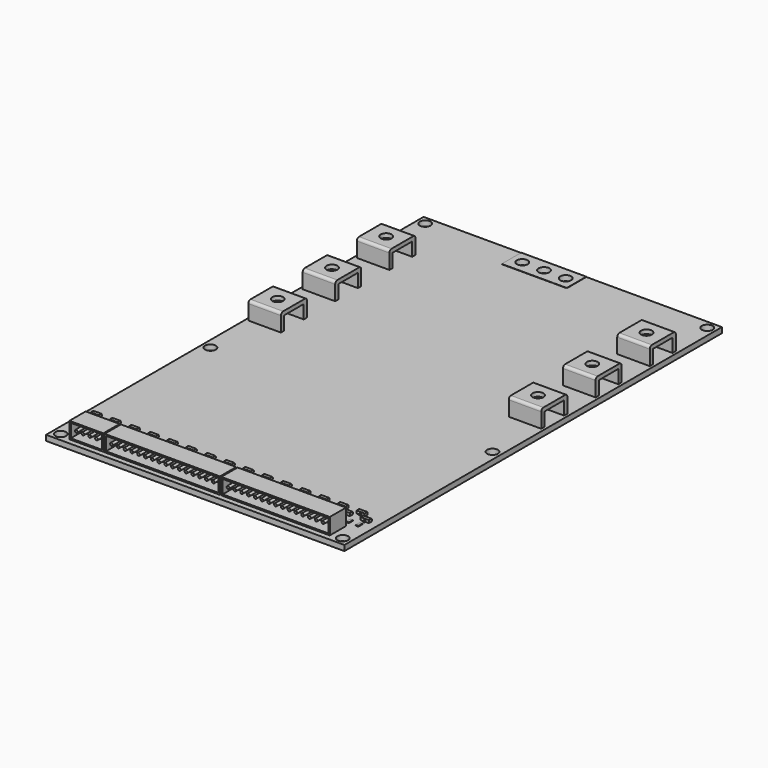
from build123d import *

# Parameters (mm, degrees)
F0_W      = 110
F0_H      = 174
F1_DEPTH  = 2
F3_D      = 4
F4_W      = 3
F4_H      = 1.2
F5_DEPTH  = 1
F6_W      = 0.45
F6_H      = 0.5
F7_DEPTH  = 0.5
F4_W_2    = 1
F8_DEPTH  = 0.25
F6_W_2    = 1
F6_H_2    = 1.2
F6_H_3    = 0.4
F9_DEPTH  = 0.25
F10_W     = 12.5
F10_H     = 7.5
F11_DEPTH = 6
F10_W_2   = 42.5
F10_W_3   = 40
F12_W     = 12
F12_H     = 12
F12_R     = 2
F13_DEPTH = 6.5
F14_W     = 9
F14_H     = 5
F15_DEPTH = 109.001
F16_R     = 1
F16_2_R   = 1
F16_3_R   = 1
F16_4_R   = 1
F16_5_R   = 1
F16_6_R   = 1
F17_W     = 24
F17_H     = 9
F17_R     = 2
F18_DEPTH = 0.1
F19_D     = 4.5
F19_DEPTH = 2.001
F20_W     = 39
F20_H     = 5
F20_R     = 0.5
F20_W_2   = 41.5
F20_W_3   = 11.5
F21_DEPTH = 5


with BuildPart() as f1:
    # F0 (on Top) → F1 (new body)
    with BuildSketch(Plane.XY):
        with Locations((25.1564069837, 32.1259858906)):
            Rectangle(F0_W, F0_H)
    extrude(amount=F1_DEPTH)

    # F3 (through all)
    with Locations(Plane.XY.offset(2)):
        with Locations((77.1564069837, 116.1259858906), (-26.8435930163, 116.1259858906), (-26.8435930163, 17.1259858906), (77.1564069837, 17.1259858906), (77.1564069837, -51.8740141094), (-26.8435930163, -51.8740141094)):
            Hole(F3_D / 2)

    # F19 (through all, one way)
    with BuildSketch(Plane.XY.offset(2)):
        with Locations((10.1564069837, 114.6259858906), (18.1564069837, 114.6259858906), (26.1564069837, 114.6259858906)):
            Circle(F19_D / 2)
    extrude(amount=-F19_DEPTH, mode=Mode.SUBTRACT)


with BuildPart() as f5:
    # F4 (on face) → F5 (new body)
    with BuildSketch(Plane.XY.offset(2)):
        with Locations((40.6564069837, -39.2740141094)):
            Rectangle(F4_W, F4_H)
    extrude(amount=F5_DEPTH)


with BuildPart() as f5b:
    # F4 (on face) → F5, piece 2 (new body)
    with BuildSketch(Plane.XY.offset(2)):
        with Locations((75.6564069837, -39.2740141094)):
            Rectangle(F4_W, F4_H)
    extrude(amount=F5_DEPTH)


with BuildPart() as f5c:
    # F4 (on face) → F5, piece 3 (new body)
    with BuildSketch(Plane.XY.offset(2)):
        with Locations((9.1564069837, -36.7740141094)):
            Rectangle(F4_W, F4_H)
    extrude(amount=F5_DEPTH)


with BuildPart() as f5d:
    # F4 (on face) → F5, piece 4 (new body)
    with BuildSketch(Plane.XY.offset(2)):
        with Locations((-11.8435930163, -36.7740141094)):
            Rectangle(F4_W, F4_H)
    extrude(amount=F5_DEPTH)


with BuildPart() as f5e:
    # F4 (on face) → F5, piece 5 (new body)
    with BuildSketch(Plane.XY.offset(2)):
        with Locations((23.1564069837, -36.7740141094)):
            Rectangle(F4_W, F4_H)
    extrude(amount=F5_DEPTH)


with BuildPart() as f5f:
    # F4 (on face) → F5, piece 6 (new body)
    with BuildSketch(Plane.XY.offset(2)):
        with Locations((-18.8435930163, -36.7740141094)):
            Rectangle(F4_W, F4_H)
    extrude(amount=F5_DEPTH)


with BuildPart() as f5g:
    # F4 (on face) → F5, piece 7 (new body)
    with BuildSketch(Plane.XY.offset(2)):
        with Locations((-1.3435930163, -39.2740141094)):
            Rectangle(F4_W, F4_H)
    extrude(amount=F5_DEPTH)


with BuildPart() as f5h:
    # F4 (on face) → F5, piece 8 (new body)
    with BuildSketch(Plane.XY.offset(2)):
        with Locations((12.6564069837, -39.2740141094)):
            Rectangle(F4_W, F4_H)
    extrude(amount=F5_DEPTH)


with BuildPart() as f5i:
    # F4 (on face) → F5, piece 9 (new body)
    with BuildSketch(Plane.XY.offset(2)):
        with Locations((51.1564069837, -36.7740141094)):
            Rectangle(F4_W, F4_H)
    extrude(amount=F5_DEPTH)


with BuildPart() as f5j:
    # F4 (on face) → F5, piece 10 (new body)
    with BuildSketch(Plane.XY.offset(2)):
        with Locations((72.1564069837, -36.7740141094)):
            Rectangle(F4_W, F4_H)
    extrude(amount=F5_DEPTH)


with BuildPart() as f5k:
    # F4 (on face) → F5, piece 11 (new body)
    with BuildSketch(Plane.XY.offset(2)):
        with Locations((-15.3435930163, -39.2740141094)):
            Rectangle(F4_W, F4_H)
    extrude(amount=F5_DEPTH)


with BuildPart() as f5l:
    # F4 (on face) → F5, piece 12 (new body)
    with BuildSketch(Plane.XY.offset(2)):
        with Locations((54.6564069837, -39.2740141094)):
            Rectangle(F4_W, F4_H)
    extrude(amount=F5_DEPTH)


with BuildPart() as f5m:
    # F4 (on face) → F5, piece 13 (new body)
    with BuildSketch(Plane.XY.offset(2)):
        with Locations((68.6564069837, -39.2740141094)):
            Rectangle(F4_W, F4_H)
    extrude(amount=F5_DEPTH)


with BuildPart() as f5n:
    # F4 (on face) → F5, piece 14 (new body)
    with BuildSketch(Plane.XY.offset(2)):
        with Locations((26.6564069837, -39.2740141094)):
            Rectangle(F4_W, F4_H)
    extrude(amount=F5_DEPTH)


with BuildPart() as f5o:
    # F4 (on face) → F5, piece 15 (new body)
    with BuildSketch(Plane.XY.offset(2)):
        with Locations((44.1564069837, -36.7740141094)):
            Rectangle(F4_W, F4_H)
    extrude(amount=F5_DEPTH)


with BuildPart() as f5p:
    # F4 (on face) → F5, piece 16 (new body)
    with BuildSketch(Plane.XY.offset(2)):
        with Locations((37.1564069837, -36.7740141094)):
            Rectangle(F4_W, F4_H)
    extrude(amount=F5_DEPTH)


with BuildPart() as f5q:
    # F4 (on face) → F5, piece 17 (new body)
    with BuildSketch(Plane.XY.offset(2)):
        with Locations((-22.3435930163, -39.2740141094)):
            Rectangle(F4_W, F4_H)
    extrude(amount=F5_DEPTH)


with BuildPart() as f5r:
    # F4 (on face) → F5, piece 18 (new body)
    with BuildSketch(Plane.XY.offset(2)):
        with Locations((5.6564069837, -39.2740141094)):
            Rectangle(F4_W, F4_H)
    extrude(amount=F5_DEPTH)


with BuildPart() as f5s:
    # F4 (on face) → F5, piece 19 (new body)
    with BuildSketch(Plane.XY.offset(2)):
        with Locations((16.1564069837, -36.7740141094)):
            Rectangle(F4_W, F4_H)
    extrude(amount=F5_DEPTH)


with BuildPart() as f5t:
    # F4 (on face) → F5, piece 20 (new body)
    with BuildSketch(Plane.XY.offset(2)):
        with Locations((-4.8435930163, -36.7740141094)):
            Rectangle(F4_W, F4_H)
    extrude(amount=F5_DEPTH)


with BuildPart() as f5u:
    # F4 (on face) → F5, piece 21 (new body)
    with BuildSketch(Plane.XY.offset(2)):
        with Locations((33.6564069837, -39.2740141094)):
            Rectangle(F4_W, F4_H)
    extrude(amount=F5_DEPTH)


with BuildPart() as f5v:
    # F4 (on face) → F5, piece 22 (new body)
    with BuildSketch(Plane.XY.offset(2)):
        with Locations((47.6564069837, -39.2740141094)):
            Rectangle(F4_W, F4_H)
    extrude(amount=F5_DEPTH)


with BuildPart() as f5w:
    # F4 (on face) → F5, piece 23 (new body)
    with BuildSketch(Plane.XY.offset(2)):
        with Locations((61.6564069837, -39.2740141094)):
            Rectangle(F4_W, F4_H)
    extrude(amount=F5_DEPTH)


with BuildPart() as f5x:
    # F4 (on face) → F5, piece 24 (new body)
    with BuildSketch(Plane.XY.offset(2)):
        with Locations((19.6564069837, -39.2740141094)):
            Rectangle(F4_W, F4_H)
    extrude(amount=F5_DEPTH)


with BuildPart() as f5y:
    # F4 (on face) → F5, piece 25 (new body)
    with BuildSketch(Plane.XY.offset(2)):
        with Locations((58.1564069837, -36.7740141094)):
            Rectangle(F4_W, F4_H)
    extrude(amount=F5_DEPTH)


with BuildPart() as f5z:
    # F4 (on face) → F5, piece 26 (new body)
    with BuildSketch(Plane.XY.offset(2)):
        with Locations((65.1564069837, -36.7740141094)):
            Rectangle(F4_W, F4_H)
    extrude(amount=F5_DEPTH)


with BuildPart() as f5ba:
    # F4 (on face) → F5, piece 27 (new body)
    with BuildSketch(Plane.XY.offset(2)):
        with Locations((-8.3435930163, -39.2740141094)):
            Rectangle(F4_W, F4_H)
    extrude(amount=F5_DEPTH)


with BuildPart() as f5bb:
    # F4 (on face) → F5, piece 28 (new body)
    with BuildSketch(Plane.XY.offset(2)):
        with Locations((-25.8435930163, -36.7740141094)):
            Rectangle(F4_W, F4_H)
    extrude(amount=F5_DEPTH)


with BuildPart() as f5bc:
    # F4 (on face) → F5, piece 29 (new body)
    with BuildSketch(Plane.XY.offset(2)):
        with Locations((30.1564069837, -36.7740141094)):
            Rectangle(F4_W, F4_H)
    extrude(amount=F5_DEPTH)


with BuildPart() as f5bd:
    # F4 (on face) → F5, piece 30 (new body)
    with BuildSketch(Plane.XY.offset(2)):
        with Locations((2.1564069837, -36.7740141094)):
            Rectangle(F4_W, F4_H)
    extrude(amount=F5_DEPTH)


with BuildPart() as f7:
    # F6 (on face) → F7 (new body)
    with BuildSketch(Plane.XY.offset(2)):
        with Locations((12.6564069837, -40.1240141094)):
            Rectangle(F6_W, F6_H)
        with Locations((-0.3435930163, -38.4240141094)):
            Rectangle(F6_W, F6_H)
        with Locations((52.1564069837, -35.9240141094)):
            Rectangle(F6_W, F6_H)
        with Locations((74.6564069837, -38.4240141094)):
            Rectangle(F6_W, F6_H)
        with Locations((67.6564069837, -38.4240141094)):
            Rectangle(F6_W, F6_H)
        with Locations((25.6564069837, -38.4240141094)):
            Rectangle(F6_W, F6_H)
        with Locations((71.1564069837, -35.9240141094)):
            Rectangle(F6_W, F6_H)
        with Locations((-15.3435930163, -40.1240141094)):
            Rectangle(F6_W, F6_H)
        with Locations((15.1564069837, -35.9240141094)):
            Rectangle(F6_W, F6_H)
        with Locations((-23.3435930163, -38.4240141094)):
            Rectangle(F6_W, F6_H)
        with Locations((13.6564069837, -38.4240141094)):
            Rectangle(F6_W, F6_H)
        with Locations((-5.8435930163, -35.9240141094)):
            Rectangle(F6_W, F6_H)
        with Locations((27.6564069837, -38.4240141094)):
            Rectangle(F6_W, F6_H)
        with Locations((43.1564069837, -35.9240141094)):
            Rectangle(F6_W, F6_H)
        with Locations((41.6564069837, -38.4240141094)):
            Rectangle(F6_W, F6_H)
        with Locations((-10.8435930163, -35.9240141094)):
            Rectangle(F6_W, F6_H)
        with Locations((-19.8435930163, -35.9240141094)):
            Rectangle(F6_W, F6_H)
        with Locations((44.1564069837, -37.6240141094)):
            Rectangle(F6_W, F6_H)
        with Locations((20.6564069837, -38.4240141094)):
            Rectangle(F6_W, F6_H)
        with Locations((46.6564069837, -38.4240141094)):
            Rectangle(F6_W, F6_H)
        with Locations((-2.3435930163, -38.4240141094)):
            Rectangle(F6_W, F6_H)
        with Locations((-8.3435930163, -40.1240141094)):
            Rectangle(F6_W, F6_H)
        with Locations((-18.8435930163, -37.6240141094)):
            Rectangle(F6_W, F6_H)
        with Locations((-1.3435930163, -40.1240141094)):
            Rectangle(F6_W, F6_H)
        with Locations((32.6564069837, -38.4240141094)):
            Rectangle(F6_W, F6_H)
        with Locations((66.1564069837, -35.9240141094)):
            Rectangle(F6_W, F6_H)
        with Locations((16.1564069837, -37.6240141094)):
            Rectangle(F6_W, F6_H)
        with Locations((26.6564069837, -40.1240141094)):
            Rectangle(F6_W, F6_H)
        with Locations((50.1564069837, -35.9240141094)):
            Rectangle(F6_W, F6_H)
        with Locations((24.1564069837, -35.9240141094)):
            Rectangle(F6_W, F6_H)
        with Locations((36.1564069837, -35.9240141094)):
            Rectangle(F6_W, F6_H)
        with Locations((37.1564069837, -37.6240141094)):
            Rectangle(F6_W, F6_H)
        with Locations((34.6564069837, -38.4240141094)):
            Rectangle(F6_W, F6_H)
        with Locations((53.6564069837, -38.4240141094)):
            Rectangle(F6_W, F6_H)
        with Locations((55.6564069837, -38.4240141094)):
            Rectangle(F6_W, F6_H)
        with Locations((-3.8435930163, -35.9240141094)):
            Rectangle(F6_W, F6_H)
        with Locations((17.1564069837, -35.9240141094)):
            Rectangle(F6_W, F6_H)
        with Locations((-21.3435930163, -38.4240141094)):
            Rectangle(F6_W, F6_H)
        with Locations((54.6564069837, -40.1240141094)):
            Rectangle(F6_W, F6_H)
        with Locations((68.6564069837, -40.1240141094)):
            Rectangle(F6_W, F6_H)
        with Locations((-7.3435930163, -38.4240141094)):
            Rectangle(F6_W, F6_H)
        with Locations((40.6564069837, -40.1240141094)):
            Rectangle(F6_W, F6_H)
        with Locations((62.6564069837, -38.4240141094)):
            Rectangle(F6_W, F6_H)
        with Locations((29.1564069837, -35.9240141094)):
            Rectangle(F6_W, F6_H)
        with Locations((-4.8435930163, -37.6240141094)):
            Rectangle(F6_W, F6_H)
        with Locations((64.1564069837, -35.9240141094)):
            Rectangle(F6_W, F6_H)
        with Locations((8.1564069837, -35.9240141094)):
            Rectangle(F6_W, F6_H)
        with Locations((48.6564069837, -38.4240141094)):
            Rectangle(F6_W, F6_H)
        with Locations((-17.8435930163, -35.9240141094)):
            Rectangle(F6_W, F6_H)
        with Locations((38.1564069837, -35.9240141094)):
            Rectangle(F6_W, F6_H)
        with Locations((69.6564069837, -38.4240141094)):
            Rectangle(F6_W, F6_H)
        with Locations((10.1564069837, -35.9240141094)):
            Rectangle(F6_W, F6_H)
        with Locations((-26.8435930163, -35.9240141094)):
            Rectangle(F6_W, F6_H)
        with Locations((57.1564069837, -35.9240141094)):
            Rectangle(F6_W, F6_H)
        with Locations((76.6564069837, -38.4240141094)):
            Rectangle(F6_W, F6_H)
        with Locations((39.6564069837, -38.4240141094)):
            Rectangle(F6_W, F6_H)
        with Locations((65.1564069837, -37.6240141094)):
            Rectangle(F6_W, F6_H)
        with Locations((11.6564069837, -38.4240141094)):
            Rectangle(F6_W, F6_H)
        with Locations((23.1564069837, -37.6240141094)):
            Rectangle(F6_W, F6_H)
        with Locations((1.1564069837, -35.9240141094)):
            Rectangle(F6_W, F6_H)
        with Locations((51.1564069837, -37.6240141094)):
            Rectangle(F6_W, F6_H)
        with Locations((22.1564069837, -35.9240141094)):
            Rectangle(F6_W, F6_H)
        with Locations((-12.8435930163, -35.9240141094)):
            Rectangle(F6_W, F6_H)
        with Locations((9.1564069837, -37.6240141094)):
            Rectangle(F6_W, F6_H)
        with Locations((19.6564069837, -40.1240141094)):
            Rectangle(F6_W, F6_H)
        with Locations((6.6564069837, -38.4240141094)):
            Rectangle(F6_W, F6_H)
        with Locations((-16.3435930163, -38.4240141094)):
            Rectangle(F6_W, F6_H)
        with Locations((-22.3435930163, -40.1240141094)):
            Rectangle(F6_W, F6_H)
        with Locations((-14.3435930163, -38.4240141094)):
            Rectangle(F6_W, F6_H)
        with Locations((75.6564069837, -40.1240141094)):
            Rectangle(F6_W, F6_H)
        with Locations((73.1564069837, -35.9240141094)):
            Rectangle(F6_W, F6_H)
        with Locations((2.1564069837, -37.6240141094)):
            Rectangle(F6_W, F6_H)
        with Locations((45.1564069837, -35.9240141094)):
            Rectangle(F6_W, F6_H)
        with Locations((-24.8435930163, -35.9240141094)):
            Rectangle(F6_W, F6_H)
        with Locations((58.1564069837, -37.6240141094)):
            Rectangle(F6_W, F6_H)
        with Locations((18.6564069837, -38.4240141094)):
            Rectangle(F6_W, F6_H)
        with Locations((47.6564069837, -40.1240141094)):
            Rectangle(F6_W, F6_H)
        with Locations((33.6564069837, -40.1240141094)):
            Rectangle(F6_W, F6_H)
        with Locations((31.1564069837, -35.9240141094)):
            Rectangle(F6_W, F6_H)
        with Locations((30.1564069837, -37.6240141094)):
            Rectangle(F6_W, F6_H)
        with Locations((-25.8435930163, -37.6240141094)):
            Rectangle(F6_W, F6_H)
        with Locations((60.6564069837, -38.4240141094)):
            Rectangle(F6_W, F6_H)
        with Locations((-9.3435930163, -38.4240141094)):
            Rectangle(F6_W, F6_H)
        with Locations((61.6564069837, -40.1240141094)):
            Rectangle(F6_W, F6_H)
        with Locations((-11.8435930163, -37.6240141094)):
            Rectangle(F6_W, F6_H)
        with Locations((3.1564069837, -35.9240141094)):
            Rectangle(F6_W, F6_H)
        with Locations((5.6564069837, -40.1240141094)):
            Rectangle(F6_W, F6_H)
        with Locations((59.1564069837, -35.9240141094)):
            Rectangle(F6_W, F6_H)
        with Locations((4.6564069837, -38.4240141094)):
            Rectangle(F6_W, F6_H)
        with Locations((72.1564069837, -37.6240141094)):
            Rectangle(F6_W, F6_H)
    extrude(amount=F7_DEPTH)


with BuildPart() as f8:
    # F4 (on face) → F8 (new body)
    with BuildSketch(Plane.XY.offset(2)):
        with Locations((-18.8435930163, -42.4740141094)):
            Rectangle(F4_W_2, F4_H)
    extrude(amount=F8_DEPTH)


with BuildPart() as f8b:
    # F4 (on face) → F8, piece 2 (new body)
    with BuildSketch(Plane.XY.offset(2)):
        with Locations((-22.3435930163, -42.4740141094)):
            Rectangle(F4_W_2, F4_H)
    extrude(amount=F8_DEPTH)


with BuildPart() as f8c:
    # F4 (on face) → F8, piece 3 (new body)
    with BuildSketch(Plane.XY.offset(2)):
        with Locations((26.6564069837, -42.4740141094)):
            Rectangle(F4_W_2, F4_H)
    extrude(amount=F8_DEPTH)


with BuildPart() as f8d:
    # F4 (on face) → F8, piece 4 (new body)
    with BuildSketch(Plane.XY.offset(2)):
        with Locations((-25.8435930163, -42.4740141094)):
            Rectangle(F4_W_2, F4_H)
    extrude(amount=F8_DEPTH)


with BuildPart() as f8e:
    # F4 (on face) → F8, piece 5 (new body)
    with BuildSketch(Plane.XY.offset(2)):
        with Locations((51.1564069837, -42.4740141094)):
            Rectangle(F4_W_2, F4_H)
    extrude(amount=F8_DEPTH)


with BuildPart() as f8f:
    # F4 (on face) → F8, piece 6 (new body)
    with BuildSketch(Plane.XY.offset(2)):
        with Locations((44.1564069837, -42.4740141094)):
            Rectangle(F4_W_2, F4_H)
    extrude(amount=F8_DEPTH)


with BuildPart() as f8g:
    # F4 (on face) → F8, piece 7 (new body)
    with BuildSketch(Plane.XY.offset(2)):
        with Locations((65.1564069837, -42.4740141094)):
            Rectangle(F4_W_2, F4_H)
    extrude(amount=F8_DEPTH)


with BuildPart() as f8h:
    # F4 (on face) → F8, piece 8 (new body)
    with BuildSketch(Plane.XY.offset(2)):
        with Locations((61.6564069837, -42.4740141094)):
            Rectangle(F4_W_2, F4_H)
    extrude(amount=F8_DEPTH)


with BuildPart() as f8i:
    # F4 (on face) → F8, piece 9 (new body)
    with BuildSketch(Plane.XY.offset(2)):
        with Locations((40.6564069837, -42.4740141094)):
            Rectangle(F4_W_2, F4_H)
    extrude(amount=F8_DEPTH)


with BuildPart() as f8j:
    # F4 (on face) → F8, piece 10 (new body)
    with BuildSketch(Plane.XY.offset(2)):
        with Locations((33.6564069837, -42.4740141094)):
            Rectangle(F4_W_2, F4_H)
    extrude(amount=F8_DEPTH)


with BuildPart() as f8k:
    # F4 (on face) → F8, piece 11 (new body)
    with BuildSketch(Plane.XY.offset(2)):
        with Locations((75.6564069837, -42.4740141094)):
            Rectangle(F4_W_2, F4_H)
    extrude(amount=F8_DEPTH)


with BuildPart() as f8l:
    # F4 (on face) → F8, piece 12 (new body)
    with BuildSketch(Plane.XY.offset(2)):
        with Locations((54.6564069837, -42.4740141094)):
            Rectangle(F4_W_2, F4_H)
    extrude(amount=F8_DEPTH)


with BuildPart() as f8m:
    # F4 (on face) → F8, piece 13 (new body)
    with BuildSketch(Plane.XY.offset(2)):
        with Locations((47.6564069837, -42.4740141094)):
            Rectangle(F4_W_2, F4_H)
    extrude(amount=F8_DEPTH)


with BuildPart() as f8n:
    # F4 (on face) → F8, piece 14 (new body)
    with BuildSketch(Plane.XY.offset(2)):
        with Locations((-15.3435930163, -42.4740141094)):
            Rectangle(F4_W_2, F4_H)
    extrude(amount=F8_DEPTH)


with BuildPart() as f8o:
    # F4 (on face) → F8, piece 15 (new body)
    with BuildSketch(Plane.XY.offset(2)):
        with Locations((12.6564069837, -42.4740141094)):
            Rectangle(F4_W_2, F4_H)
    extrude(amount=F8_DEPTH)


with BuildPart() as f8p:
    # F4 (on face) → F8, piece 16 (new body)
    with BuildSketch(Plane.XY.offset(2)):
        with Locations((-8.3435930163, -42.4740141094)):
            Rectangle(F4_W_2, F4_H)
    extrude(amount=F8_DEPTH)


with BuildPart() as f8q:
    # F4 (on face) → F8, piece 17 (new body)
    with BuildSketch(Plane.XY.offset(2)):
        with Locations((-1.3435930163, -42.4740141094)):
            Rectangle(F4_W_2, F4_H)
    extrude(amount=F8_DEPTH)


with BuildPart() as f8r:
    # F4 (on face) → F8, piece 18 (new body)
    with BuildSketch(Plane.XY.offset(2)):
        with Locations((19.6564069837, -42.4740141094)):
            Rectangle(F4_W_2, F4_H)
    extrude(amount=F8_DEPTH)


with BuildPart() as f8s:
    # F4 (on face) → F8, piece 19 (new body)
    with BuildSketch(Plane.XY.offset(2)):
        with Locations((5.6564069837, -42.4740141094)):
            Rectangle(F4_W_2, F4_H)
    extrude(amount=F8_DEPTH)


with BuildPart() as f8t:
    # F4 (on face) → F8, piece 20 (new body)
    with BuildSketch(Plane.XY.offset(2)):
        with Locations((72.1564069837, -42.4740141094)):
            Rectangle(F4_W_2, F4_H)
    extrude(amount=F8_DEPTH)


with BuildPart() as f8u:
    # F4 (on face) → F8, piece 21 (new body)
    with BuildSketch(Plane.XY.offset(2)):
        with Locations((58.1564069837, -42.4740141094)):
            Rectangle(F4_W_2, F4_H)
    extrude(amount=F8_DEPTH)


with BuildPart() as f8v:
    # F4 (on face) → F8, piece 22 (new body)
    with BuildSketch(Plane.XY.offset(2)):
        with Locations((30.1564069837, -42.4740141094)):
            Rectangle(F4_W_2, F4_H)
    extrude(amount=F8_DEPTH)


with BuildPart() as f8w:
    # F4 (on face) → F8, piece 23 (new body)
    with BuildSketch(Plane.XY.offset(2)):
        with Locations((9.1564069837, -42.4740141094)):
            Rectangle(F4_W_2, F4_H)
    extrude(amount=F8_DEPTH)


with BuildPart() as f8x:
    # F4 (on face) → F8, piece 24 (new body)
    with BuildSketch(Plane.XY.offset(2)):
        with Locations((-11.8435930163, -42.4740141094)):
            Rectangle(F4_W_2, F4_H)
    extrude(amount=F8_DEPTH)


with BuildPart() as f8y:
    # F4 (on face) → F8, piece 25 (new body)
    with BuildSketch(Plane.XY.offset(2)):
        with Locations((-4.8435930163, -42.4740141094)):
            Rectangle(F4_W_2, F4_H)
    extrude(amount=F8_DEPTH)


with BuildPart() as f8z:
    # F4 (on face) → F8, piece 26 (new body)
    with BuildSketch(Plane.XY.offset(2)):
        with Locations((16.1564069837, -42.4740141094)):
            Rectangle(F4_W_2, F4_H)
    extrude(amount=F8_DEPTH)


with BuildPart() as f8ba:
    # F4 (on face) → F8, piece 27 (new body)
    with BuildSketch(Plane.XY.offset(2)):
        with Locations((23.1564069837, -42.4740141094)):
            Rectangle(F4_W_2, F4_H)
    extrude(amount=F8_DEPTH)


with BuildPart() as f8bb:
    # F4 (on face) → F8, piece 28 (new body)
    with BuildSketch(Plane.XY.offset(2)):
        with Locations((2.1564069837, -42.4740141094)):
            Rectangle(F4_W_2, F4_H)
    extrude(amount=F8_DEPTH)


with BuildPart() as f8bc:
    # F4 (on face) → F8, piece 29 (new body)
    with BuildSketch(Plane.XY.offset(2)):
        with Locations((68.6564069837, -42.4740141094)):
            Rectangle(F4_W_2, F4_H)
    extrude(amount=F8_DEPTH)


with BuildPart() as f8bd:
    # F4 (on face) → F8, piece 30 (new body)
    with BuildSketch(Plane.XY.offset(2)):
        with Locations((37.1564069837, -42.4740141094)):
            Rectangle(F4_W_2, F4_H)
    extrude(amount=F8_DEPTH)


with BuildPart() as f8be:
    # F6 (on face) → F8, piece 31 (new body)
    with BuildSketch(Plane.XY.offset(2)):
        with Locations((2.1564069837, -42.4740141094)):
            Rectangle(F6_W_2, F6_H_2)
    extrude(amount=F8_DEPTH)


with BuildPart() as f8bf:
    # F6 (on face) → F8, piece 32 (new body)
    with BuildSketch(Plane.XY.offset(2)):
        with Locations((33.6564069837, -42.4740141094)):
            Rectangle(F6_W_2, F6_H_2)
    extrude(amount=F8_DEPTH)


with BuildPart() as f8bg:
    # F6 (on face) → F8, piece 33 (new body)
    with BuildSketch(Plane.XY.offset(2)):
        with Locations((-1.3435930163, -42.4740141094)):
            Rectangle(F6_W_2, F6_H_2)
    extrude(amount=F8_DEPTH)


with BuildPart() as f8bh:
    # F6 (on face) → F8, piece 34 (new body)
    with BuildSketch(Plane.XY.offset(2)):
        with Locations((23.1564069837, -42.4740141094)):
            Rectangle(F6_W_2, F6_H_2)
    extrude(amount=F8_DEPTH)


with BuildPart() as f8bi:
    # F6 (on face) → F8, piece 35 (new body)
    with BuildSketch(Plane.XY.offset(2)):
        with Locations((16.1564069837, -42.4740141094)):
            Rectangle(F6_W_2, F6_H_2)
    extrude(amount=F8_DEPTH)


with BuildPart() as f8bj:
    # F6 (on face) → F8, piece 36 (new body)
    with BuildSketch(Plane.XY.offset(2)):
        with Locations((5.6564069837, -42.4740141094)):
            Rectangle(F6_W_2, F6_H_2)
    extrude(amount=F8_DEPTH)


with BuildPart() as f8bk:
    # F6 (on face) → F8, piece 37 (new body)
    with BuildSketch(Plane.XY.offset(2)):
        with Locations((54.6564069837, -42.4740141094)):
            Rectangle(F6_W_2, F6_H_2)
    extrude(amount=F8_DEPTH)


with BuildPart() as f8bl:
    # F6 (on face) → F8, piece 38 (new body)
    with BuildSketch(Plane.XY.offset(2)):
        with Locations((30.1564069837, -42.4740141094)):
            Rectangle(F6_W_2, F6_H_2)
    extrude(amount=F8_DEPTH)


with BuildPart() as f8bm:
    # F6 (on face) → F8, piece 39 (new body)
    with BuildSketch(Plane.XY.offset(2)):
        with Locations((-22.3435930163, -42.4740141094)):
            Rectangle(F6_W_2, F6_H_2)
    extrude(amount=F8_DEPTH)


with BuildPart() as f8bn:
    # F6 (on face) → F8, piece 40 (new body)
    with BuildSketch(Plane.XY.offset(2)):
        with Locations((68.6564069837, -42.4740141094)):
            Rectangle(F6_W_2, F6_H_2)
    extrude(amount=F8_DEPTH)


with BuildPart() as f8bo:
    # F6 (on face) → F8, piece 41 (new body)
    with BuildSketch(Plane.XY.offset(2)):
        with Locations((-18.8435930163, -42.4740141094)):
            Rectangle(F6_W_2, F6_H_2)
    extrude(amount=F8_DEPTH)


with BuildPart() as f8bp:
    # F6 (on face) → F8, piece 42 (new body)
    with BuildSketch(Plane.XY.offset(2)):
        with Locations((-15.3435930163, -42.4740141094)):
            Rectangle(F6_W_2, F6_H_2)
    extrude(amount=F8_DEPTH)


with BuildPart() as f8bq:
    # F6 (on face) → F8, piece 43 (new body)
    with BuildSketch(Plane.XY.offset(2)):
        with Locations((37.1564069837, -42.4740141094)):
            Rectangle(F6_W_2, F6_H_2)
    extrude(amount=F8_DEPTH)


with BuildPart() as f8br:
    # F6 (on face) → F8, piece 44 (new body)
    with BuildSketch(Plane.XY.offset(2)):
        with Locations((-25.8435930163, -42.4740141094)):
            Rectangle(F6_W_2, F6_H_2)
    extrude(amount=F8_DEPTH)


with BuildPart() as f8bs:
    # F6 (on face) → F8, piece 45 (new body)
    with BuildSketch(Plane.XY.offset(2)):
        with Locations((19.6564069837, -42.4740141094)):
            Rectangle(F6_W_2, F6_H_2)
    extrude(amount=F8_DEPTH)


with BuildPart() as f8bt:
    # F6 (on face) → F8, piece 46 (new body)
    with BuildSketch(Plane.XY.offset(2)):
        with Locations((26.6564069837, -42.4740141094)):
            Rectangle(F6_W_2, F6_H_2)
    extrude(amount=F8_DEPTH)


with BuildPart() as f8bu:
    # F6 (on face) → F8, piece 47 (new body)
    with BuildSketch(Plane.XY.offset(2)):
        with Locations((75.6564069837, -42.4740141094)):
            Rectangle(F6_W_2, F6_H_2)
    extrude(amount=F8_DEPTH)


with BuildPart() as f8bv:
    # F6 (on face) → F8, piece 48 (new body)
    with BuildSketch(Plane.XY.offset(2)):
        with Locations((-4.8435930163, -42.4740141094)):
            Rectangle(F6_W_2, F6_H_2)
    extrude(amount=F8_DEPTH)


with BuildPart() as f8bw:
    # F6 (on face) → F8, piece 49 (new body)
    with BuildSketch(Plane.XY.offset(2)):
        with Locations((58.1564069837, -42.4740141094)):
            Rectangle(F6_W_2, F6_H_2)
    extrude(amount=F8_DEPTH)


with BuildPart() as f8bx:
    # F6 (on face) → F8, piece 50 (new body)
    with BuildSketch(Plane.XY.offset(2)):
        with Locations((40.6564069837, -42.4740141094)):
            Rectangle(F6_W_2, F6_H_2)
    extrude(amount=F8_DEPTH)


with BuildPart() as f8by:
    # F6 (on face) → F8, piece 51 (new body)
    with BuildSketch(Plane.XY.offset(2)):
        with Locations((72.1564069837, -42.4740141094)):
            Rectangle(F6_W_2, F6_H_2)
    extrude(amount=F8_DEPTH)


with BuildPart() as f8bz:
    # F6 (on face) → F8, piece 52 (new body)
    with BuildSketch(Plane.XY.offset(2)):
        with Locations((9.1564069837, -42.4740141094)):
            Rectangle(F6_W_2, F6_H_2)
    extrude(amount=F8_DEPTH)


with BuildPart() as f8ca:
    # F6 (on face) → F8, piece 53 (new body)
    with BuildSketch(Plane.XY.offset(2)):
        with Locations((65.1564069837, -42.4740141094)):
            Rectangle(F6_W_2, F6_H_2)
    extrude(amount=F8_DEPTH)


with BuildPart() as f8cb:
    # F6 (on face) → F8, piece 54 (new body)
    with BuildSketch(Plane.XY.offset(2)):
        with Locations((44.1564069837, -42.4740141094)):
            Rectangle(F6_W_2, F6_H_2)
    extrude(amount=F8_DEPTH)


with BuildPart() as f8cc:
    # F6 (on face) → F8, piece 55 (new body)
    with BuildSketch(Plane.XY.offset(2)):
        with Locations((12.6564069837, -42.4740141094)):
            Rectangle(F6_W_2, F6_H_2)
    extrude(amount=F8_DEPTH)


with BuildPart() as f8cd:
    # F6 (on face) → F8, piece 56 (new body)
    with BuildSketch(Plane.XY.offset(2)):
        with Locations((61.6564069837, -42.4740141094)):
            Rectangle(F6_W_2, F6_H_2)
    extrude(amount=F8_DEPTH)


with BuildPart() as f8ce:
    # F6 (on face) → F8, piece 57 (new body)
    with BuildSketch(Plane.XY.offset(2)):
        with Locations((-11.8435930163, -42.4740141094)):
            Rectangle(F6_W_2, F6_H_2)
    extrude(amount=F8_DEPTH)


with BuildPart() as f8cf:
    # F6 (on face) → F8, piece 58 (new body)
    with BuildSketch(Plane.XY.offset(2)):
        with Locations((47.6564069837, -42.4740141094)):
            Rectangle(F6_W_2, F6_H_2)
    extrude(amount=F8_DEPTH)


with BuildPart() as f8cg:
    # F6 (on face) → F8, piece 59 (new body)
    with BuildSketch(Plane.XY.offset(2)):
        with Locations((51.1564069837, -42.4740141094)):
            Rectangle(F6_W_2, F6_H_2)
    extrude(amount=F8_DEPTH)


with BuildPart() as f8ch:
    # F6 (on face) → F8, piece 60 (new body)
    with BuildSketch(Plane.XY.offset(2)):
        with Locations((-8.3435930163, -42.4740141094)):
            Rectangle(F6_W_2, F6_H_2)
    extrude(amount=F8_DEPTH)


with BuildPart() as f9:
    # F6 (on face) → F9 (new body)
    with BuildSketch(Plane.XY.offset(2)):
        with Locations((54.6564069837, -41.6740141094)):
            Rectangle(F6_W_2, F6_H_3)
    extrude(amount=F9_DEPTH)


with BuildPart() as f9b:
    # F6 (on face) → F9, piece 2 (new body)
    with BuildSketch(Plane.XY.offset(2)):
        with Locations((26.6564069837, -41.6740141094)):
            Rectangle(F6_W_2, F6_H_3)
    extrude(amount=F9_DEPTH)


with BuildPart() as f9c:
    # F6 (on face) → F9, piece 3 (new body)
    with BuildSketch(Plane.XY.offset(2)):
        with Locations((-1.3435930163, -41.6740141094)):
            Rectangle(F6_W_2, F6_H_3)
    extrude(amount=F9_DEPTH)


with BuildPart() as f9d:
    # F6 (on face) → F9, piece 4 (new body)
    with BuildSketch(Plane.XY.offset(2)):
        with Locations((33.6564069837, -41.6740141094)):
            Rectangle(F6_W_2, F6_H_3)
    extrude(amount=F9_DEPTH)


with BuildPart() as f9e:
    # F6 (on face) → F9, piece 5 (new body)
    with BuildSketch(Plane.XY.offset(2)):
        with Locations((37.1564069837, -41.6740141094)):
            Rectangle(F6_W_2, F6_H_3)
    extrude(amount=F9_DEPTH)


with BuildPart() as f9f:
    # F6 (on face) → F9, piece 6 (new body)
    with BuildSketch(Plane.XY.offset(2)):
        with Locations((23.1564069837, -41.6740141094)):
            Rectangle(F6_W_2, F6_H_3)
    extrude(amount=F9_DEPTH)


with BuildPart() as f9g:
    # F6 (on face) → F9, piece 7 (new body)
    with BuildSketch(Plane.XY.offset(2)):
        with Locations((-8.3435930163, -41.6740141094)):
            Rectangle(F6_W_2, F6_H_3)
    extrude(amount=F9_DEPTH)


with BuildPart() as f9h:
    # F6 (on face) → F9, piece 8 (new body)
    with BuildSketch(Plane.XY.offset(2)):
        with Locations((2.1564069837, -41.6740141094)):
            Rectangle(F6_W_2, F6_H_3)
    extrude(amount=F9_DEPTH)


with BuildPart() as f9i:
    # F6 (on face) → F9, piece 9 (new body)
    with BuildSketch(Plane.XY.offset(2)):
        with Locations((40.6564069837, -41.6740141094)):
            Rectangle(F6_W_2, F6_H_3)
    extrude(amount=F9_DEPTH)


with BuildPart() as f9j:
    # F6 (on face) → F9, piece 10 (new body)
    with BuildSketch(Plane.XY.offset(2)):
        with Locations((68.6564069837, -41.6740141094)):
            Rectangle(F6_W_2, F6_H_3)
    extrude(amount=F9_DEPTH)


with BuildPart() as f9k:
    # F6 (on face) → F9, piece 11 (new body)
    with BuildSketch(Plane.XY.offset(2)):
        with Locations((5.6564069837, -41.6740141094)):
            Rectangle(F6_W_2, F6_H_3)
    extrude(amount=F9_DEPTH)


with BuildPart() as f9l:
    # F6 (on face) → F9, piece 12 (new body)
    with BuildSketch(Plane.XY.offset(2)):
        with Locations((30.1564069837, -41.6740141094)):
            Rectangle(F6_W_2, F6_H_3)
    extrude(amount=F9_DEPTH)


with BuildPart() as f9m:
    # F6 (on face) → F9, piece 13 (new body)
    with BuildSketch(Plane.XY.offset(2)):
        with Locations((58.1564069837, -41.6740141094)):
            Rectangle(F6_W_2, F6_H_3)
    extrude(amount=F9_DEPTH)


with BuildPart() as f9n:
    # F6 (on face) → F9, piece 14 (new body)
    with BuildSketch(Plane.XY.offset(2)):
        with Locations((-25.8435930163, -41.6740141094)):
            Rectangle(F6_W_2, F6_H_3)
    extrude(amount=F9_DEPTH)


with BuildPart() as f9o:
    # F6 (on face) → F9, piece 15 (new body)
    with BuildSketch(Plane.XY.offset(2)):
        with Locations((-22.3435930163, -41.6740141094)):
            Rectangle(F6_W_2, F6_H_3)
    extrude(amount=F9_DEPTH)


with BuildPart() as f9p:
    # F6 (on face) → F9, piece 16 (new body)
    with BuildSketch(Plane.XY.offset(2)):
        with Locations((61.6564069837, -41.6740141094)):
            Rectangle(F6_W_2, F6_H_3)
    extrude(amount=F9_DEPTH)


with BuildPart() as f9q:
    # F6 (on face) → F9, piece 17 (new body)
    with BuildSketch(Plane.XY.offset(2)):
        with Locations((47.6564069837, -41.6740141094)):
            Rectangle(F6_W_2, F6_H_3)
    extrude(amount=F9_DEPTH)


with BuildPart() as f9r:
    # F6 (on face) → F9, piece 18 (new body)
    with BuildSketch(Plane.XY.offset(2)):
        with Locations((-18.8435930163, -41.6740141094)):
            Rectangle(F6_W_2, F6_H_3)
    extrude(amount=F9_DEPTH)


with BuildPart() as f9s:
    # F6 (on face) → F9, piece 19 (new body)
    with BuildSketch(Plane.XY.offset(2)):
        with Locations((-15.3435930163, -41.6740141094)):
            Rectangle(F6_W_2, F6_H_3)
    extrude(amount=F9_DEPTH)


with BuildPart() as f9t:
    # F6 (on face) → F9, piece 20 (new body)
    with BuildSketch(Plane.XY.offset(2)):
        with Locations((-11.8435930163, -41.6740141094)):
            Rectangle(F6_W_2, F6_H_3)
    extrude(amount=F9_DEPTH)


with BuildPart() as f9u:
    # F6 (on face) → F9, piece 21 (new body)
    with BuildSketch(Plane.XY.offset(2)):
        with Locations((44.1564069837, -41.6740141094)):
            Rectangle(F6_W_2, F6_H_3)
    extrude(amount=F9_DEPTH)


with BuildPart() as f9v:
    # F6 (on face) → F9, piece 22 (new body)
    with BuildSketch(Plane.XY.offset(2)):
        with Locations((51.1564069837, -41.6740141094)):
            Rectangle(F6_W_2, F6_H_3)
    extrude(amount=F9_DEPTH)


with BuildPart() as f9w:
    # F6 (on face) → F9, piece 23 (new body)
    with BuildSketch(Plane.XY.offset(2)):
        with Locations((75.6564069837, -41.6740141094)):
            Rectangle(F6_W_2, F6_H_3)
    extrude(amount=F9_DEPTH)


with BuildPart() as f9x:
    # F6 (on face) → F9, piece 24 (new body)
    with BuildSketch(Plane.XY.offset(2)):
        with Locations((12.6564069837, -41.6740141094)):
            Rectangle(F6_W_2, F6_H_3)
    extrude(amount=F9_DEPTH)


with BuildPart() as f9y:
    # F6 (on face) → F9, piece 25 (new body)
    with BuildSketch(Plane.XY.offset(2)):
        with Locations((72.1564069837, -41.6740141094)):
            Rectangle(F6_W_2, F6_H_3)
    extrude(amount=F9_DEPTH)


with BuildPart() as f9z:
    # F6 (on face) → F9, piece 26 (new body)
    with BuildSketch(Plane.XY.offset(2)):
        with Locations((-4.8435930163, -41.6740141094)):
            Rectangle(F6_W_2, F6_H_3)
    extrude(amount=F9_DEPTH)


with BuildPart() as f9ba:
    # F6 (on face) → F9, piece 27 (new body)
    with BuildSketch(Plane.XY.offset(2)):
        with Locations((9.1564069837, -41.6740141094)):
            Rectangle(F6_W_2, F6_H_3)
    extrude(amount=F9_DEPTH)


with BuildPart() as f9bb:
    # F6 (on face) → F9, piece 28 (new body)
    with BuildSketch(Plane.XY.offset(2)):
        with Locations((16.1564069837, -41.6740141094)):
            Rectangle(F6_W_2, F6_H_3)
    extrude(amount=F9_DEPTH)


with BuildPart() as f9bc:
    # F6 (on face) → F9, piece 29 (new body)
    with BuildSketch(Plane.XY.offset(2)):
        with Locations((19.6564069837, -41.6740141094)):
            Rectangle(F6_W_2, F6_H_3)
    extrude(amount=F9_DEPTH)


with BuildPart() as f9bd:
    # F6 (on face) → F9, piece 30 (new body)
    with BuildSketch(Plane.XY.offset(2)):
        with Locations((65.1564069837, -41.6740141094)):
            Rectangle(F6_W_2, F6_H_3)
    extrude(amount=F9_DEPTH)


with BuildPart() as f9be:
    # F6 (on face) → F9, piece 31 (new body)
    with BuildSketch(Plane.XY.offset(2)):
        with Locations((65.1564069837, -43.2740141094)):
            Rectangle(F6_W_2, F6_H_3)
    extrude(amount=F9_DEPTH)


with BuildPart() as f9bf:
    # F6 (on face) → F9, piece 32 (new body)
    with BuildSketch(Plane.XY.offset(2)):
        with Locations((-25.8435930163, -43.2740141094)):
            Rectangle(F6_W_2, F6_H_3)
    extrude(amount=F9_DEPTH)


with BuildPart() as f9bg:
    # F6 (on face) → F9, piece 33 (new body)
    with BuildSketch(Plane.XY.offset(2)):
        with Locations((23.1564069837, -43.2740141094)):
            Rectangle(F6_W_2, F6_H_3)
    extrude(amount=F9_DEPTH)


with BuildPart() as f9bh:
    # F6 (on face) → F9, piece 34 (new body)
    with BuildSketch(Plane.XY.offset(2)):
        with Locations((72.1564069837, -43.2740141094)):
            Rectangle(F6_W_2, F6_H_3)
    extrude(amount=F9_DEPTH)


with BuildPart() as f9bi:
    # F6 (on face) → F9, piece 35 (new body)
    with BuildSketch(Plane.XY.offset(2)):
        with Locations((44.1564069837, -43.2740141094)):
            Rectangle(F6_W_2, F6_H_3)
    extrude(amount=F9_DEPTH)


with BuildPart() as f9bj:
    # F6 (on face) → F9, piece 36 (new body)
    with BuildSketch(Plane.XY.offset(2)):
        with Locations((-4.8435930163, -43.2740141094)):
            Rectangle(F6_W_2, F6_H_3)
    extrude(amount=F9_DEPTH)


with BuildPart() as f9bk:
    # F6 (on face) → F9, piece 37 (new body)
    with BuildSketch(Plane.XY.offset(2)):
        with Locations((61.6564069837, -43.2740141094)):
            Rectangle(F6_W_2, F6_H_3)
    extrude(amount=F9_DEPTH)


with BuildPart() as f9bl:
    # F6 (on face) → F9, piece 38 (new body)
    with BuildSketch(Plane.XY.offset(2)):
        with Locations((-15.3435930163, -43.2740141094)):
            Rectangle(F6_W_2, F6_H_3)
    extrude(amount=F9_DEPTH)


with BuildPart() as f9bm:
    # F6 (on face) → F9, piece 39 (new body)
    with BuildSketch(Plane.XY.offset(2)):
        with Locations((12.6564069837, -43.2740141094)):
            Rectangle(F6_W_2, F6_H_3)
    extrude(amount=F9_DEPTH)


with BuildPart() as f9bn:
    # F6 (on face) → F9, piece 40 (new body)
    with BuildSketch(Plane.XY.offset(2)):
        with Locations((19.6564069837, -43.2740141094)):
            Rectangle(F6_W_2, F6_H_3)
    extrude(amount=F9_DEPTH)


with BuildPart() as f9bo:
    # F6 (on face) → F9, piece 41 (new body)
    with BuildSketch(Plane.XY.offset(2)):
        with Locations((33.6564069837, -43.2740141094)):
            Rectangle(F6_W_2, F6_H_3)
    extrude(amount=F9_DEPTH)


with BuildPart() as f9bp:
    # F6 (on face) → F9, piece 42 (new body)
    with BuildSketch(Plane.XY.offset(2)):
        with Locations((-22.3435930163, -43.2740141094)):
            Rectangle(F6_W_2, F6_H_3)
    extrude(amount=F9_DEPTH)


with BuildPart() as f9bq:
    # F6 (on face) → F9, piece 43 (new body)
    with BuildSketch(Plane.XY.offset(2)):
        with Locations((54.6564069837, -43.2740141094)):
            Rectangle(F6_W_2, F6_H_3)
    extrude(amount=F9_DEPTH)


with BuildPart() as f9br:
    # F6 (on face) → F9, piece 44 (new body)
    with BuildSketch(Plane.XY.offset(2)):
        with Locations((58.1564069837, -43.2740141094)):
            Rectangle(F6_W_2, F6_H_3)
    extrude(amount=F9_DEPTH)


with BuildPart() as f9bs:
    # F6 (on face) → F9, piece 45 (new body)
    with BuildSketch(Plane.XY.offset(2)):
        with Locations((9.1564069837, -43.2740141094)):
            Rectangle(F6_W_2, F6_H_3)
    extrude(amount=F9_DEPTH)


with BuildPart() as f9bt:
    # F6 (on face) → F9, piece 46 (new body)
    with BuildSketch(Plane.XY.offset(2)):
        with Locations((37.1564069837, -43.2740141094)):
            Rectangle(F6_W_2, F6_H_3)
    extrude(amount=F9_DEPTH)


with BuildPart() as f9bu:
    # F6 (on face) → F9, piece 47 (new body)
    with BuildSketch(Plane.XY.offset(2)):
        with Locations((30.1564069837, -43.2740141094)):
            Rectangle(F6_W_2, F6_H_3)
    extrude(amount=F9_DEPTH)


with BuildPart() as f9bv:
    # F6 (on face) → F9, piece 48 (new body)
    with BuildSketch(Plane.XY.offset(2)):
        with Locations((68.6564069837, -43.2740141094)):
            Rectangle(F6_W_2, F6_H_3)
    extrude(amount=F9_DEPTH)


with BuildPart() as f9bw:
    # F6 (on face) → F9, piece 49 (new body)
    with BuildSketch(Plane.XY.offset(2)):
        with Locations((-1.3435930163, -43.2740141094)):
            Rectangle(F6_W_2, F6_H_3)
    extrude(amount=F9_DEPTH)


with BuildPart() as f9bx:
    # F6 (on face) → F9, piece 50 (new body)
    with BuildSketch(Plane.XY.offset(2)):
        with Locations((2.1564069837, -43.2740141094)):
            Rectangle(F6_W_2, F6_H_3)
    extrude(amount=F9_DEPTH)


with BuildPart() as f9by:
    # F6 (on face) → F9, piece 51 (new body)
    with BuildSketch(Plane.XY.offset(2)):
        with Locations((5.6564069837, -43.2740141094)):
            Rectangle(F6_W_2, F6_H_3)
    extrude(amount=F9_DEPTH)


with BuildPart() as f9bz:
    # F6 (on face) → F9, piece 52 (new body)
    with BuildSketch(Plane.XY.offset(2)):
        with Locations((-18.8435930163, -43.2740141094)):
            Rectangle(F6_W_2, F6_H_3)
    extrude(amount=F9_DEPTH)


with BuildPart() as f9ca:
    # F6 (on face) → F9, piece 53 (new body)
    with BuildSketch(Plane.XY.offset(2)):
        with Locations((40.6564069837, -43.2740141094)):
            Rectangle(F6_W_2, F6_H_3)
    extrude(amount=F9_DEPTH)


with BuildPart() as f9cb:
    # F6 (on face) → F9, piece 54 (new body)
    with BuildSketch(Plane.XY.offset(2)):
        with Locations((47.6564069837, -43.2740141094)):
            Rectangle(F6_W_2, F6_H_3)
    extrude(amount=F9_DEPTH)


with BuildPart() as f9cc:
    # F6 (on face) → F9, piece 55 (new body)
    with BuildSketch(Plane.XY.offset(2)):
        with Locations((-11.8435930163, -43.2740141094)):
            Rectangle(F6_W_2, F6_H_3)
    extrude(amount=F9_DEPTH)


with BuildPart() as f9cd:
    # F6 (on face) → F9, piece 56 (new body)
    with BuildSketch(Plane.XY.offset(2)):
        with Locations((51.1564069837, -43.2740141094)):
            Rectangle(F6_W_2, F6_H_3)
    extrude(amount=F9_DEPTH)


with BuildPart() as f9ce:
    # F6 (on face) → F9, piece 57 (new body)
    with BuildSketch(Plane.XY.offset(2)):
        with Locations((-8.3435930163, -43.2740141094)):
            Rectangle(F6_W_2, F6_H_3)
    extrude(amount=F9_DEPTH)


with BuildPart() as f9cf:
    # F6 (on face) → F9, piece 58 (new body)
    with BuildSketch(Plane.XY.offset(2)):
        with Locations((16.1564069837, -43.2740141094)):
            Rectangle(F6_W_2, F6_H_3)
    extrude(amount=F9_DEPTH)


with BuildPart() as f9cg:
    # F6 (on face) → F9, piece 59 (new body)
    with BuildSketch(Plane.XY.offset(2)):
        with Locations((26.6564069837, -43.2740141094)):
            Rectangle(F6_W_2, F6_H_3)
    extrude(amount=F9_DEPTH)


with BuildPart() as f9ch:
    # F6 (on face) → F9, piece 60 (new body)
    with BuildSketch(Plane.XY.offset(2)):
        with Locations((75.6564069837, -43.2740141094)):
            Rectangle(F6_W_2, F6_H_3)
    extrude(amount=F9_DEPTH)


with BuildPart() as f11:
    # F10 (on face) → F11 (new body)
    with BuildSketch(Plane.XY.offset(2)):
        with Locations((-16.5935930163, -49.1240141094)):
            Rectangle(F10_W, F10_H)
    extrude(amount=F11_DEPTH)


with BuildPart() as f11b:
    # F10 (on face) → F11, piece 2 (new body)
    with BuildSketch(Plane.XY.offset(2)):
        with Locations((11.4064069837, -49.1240141094)):
            Rectangle(F10_W_2, F10_H)
    extrude(amount=F11_DEPTH)


with BuildPart() as f11c:
    # F10 (on face) → F11, piece 3 (new body)
    with BuildSketch(Plane.XY.offset(2)):
        with Locations((53.1564069837, -49.1240141094)):
            Rectangle(F10_W_3, F10_H)
    extrude(amount=F11_DEPTH)


with BuildPart() as f13:
    # F12 (on face) → F13 (new body)
    with BuildSketch(Plane.XY.offset(2)):
        with Locations((-22.8435930163, 93.1259858906)):
            Rectangle(F12_W, F12_H)
        with Locations((-22.8435930163, 93.1259858906)):
            Circle(F12_R, mode=Mode.SUBTRACT)
    extrude(amount=F13_DEPTH)


with BuildPart() as f13b:
    # F12 (on face) → F13, piece 2 (new body)
    with BuildSketch(Plane.XY.offset(2)):
        with Locations((73.1564069837, 93.1259858906)):
            Rectangle(F12_W, F12_H)
        with Locations((73.1564069837, 93.1259858906)):
            Circle(F12_R, mode=Mode.SUBTRACT)
    extrude(amount=F13_DEPTH)


with BuildPart() as f13c:
    # F12 (on face) → F13, piece 3 (new body)
    with BuildSketch(Plane.XY.offset(2)):
        with Locations((73.1564069837, 68.1259858906)):
            Rectangle(F12_W, F12_H)
        with Locations((73.1564069837, 68.1259858906)):
            Circle(F12_R, mode=Mode.SUBTRACT)
    extrude(amount=F13_DEPTH)


with BuildPart() as f13d:
    # F12 (on face) → F13, piece 4 (new body)
    with BuildSketch(Plane.XY.offset(2)):
        with Locations((-22.8435930163, 68.1259858906)):
            Rectangle(F12_W, F12_H)
        with Locations((-22.8435930163, 68.1259858906)):
            Circle(F12_R, mode=Mode.SUBTRACT)
    extrude(amount=F13_DEPTH)


with BuildPart() as f13e:
    # F12 (on face) → F13, piece 5 (new body)
    with BuildSketch(Plane.XY.offset(2)):
        with Locations((-22.8435930163, 43.1259858906)):
            Rectangle(F12_W, F12_H)
        with Locations((-22.8435930163, 43.1259858906)):
            Circle(F12_R, mode=Mode.SUBTRACT)
    extrude(amount=F13_DEPTH)


with BuildPart() as f13f:
    # F12 (on face) → F13, piece 6 (new body)
    with BuildSketch(Plane.XY.offset(2)):
        with Locations((73.1564069837, 43.1259858906)):
            Rectangle(F12_W, F12_H)
        with Locations((73.1564069837, 43.1259858906)):
            Circle(F12_R, mode=Mode.SUBTRACT)
    extrude(amount=F13_DEPTH)


with BuildPart() as f15_tool:
    # F14 (on face) → F15 (new body, through all)
    with BuildSketch(Plane.YZ.offset(79.1564069837)):
        with Locations((43.1259858906, 4.5)):
            Rectangle(F14_W, F14_H)
        with Locations((68.1259858906, 4.5)):
            Rectangle(F14_W, F14_H)
        with Locations((93.1259858906, 4.5)):
            Rectangle(F14_W, F14_H)
    extrude(amount=-F15_DEPTH)


with BuildPart() as f13_1:
    add(f13.part)

    # F15: cut by f15_tool
    add(f15_tool.part, mode=Mode.SUBTRACT)

    # F16#3
    f16_3_edges = [f13_1.edges().sort_by_distance(p)[0] for p in [
        (-22.843593, 87.125986, 8.5),
        (-22.843593, 99.125986, 8.5),
    ]]
    fillet(f16_3_edges, radius=F16_3_R)


with BuildPart() as f13b_1:
    add(f13b.part)

    # F15: cut by f15_tool
    add(f15_tool.part, mode=Mode.SUBTRACT)

    # F16#6
    f16_6_edges = [f13b_1.edges().sort_by_distance(p)[0] for p in [
        (73.156407, 87.125986, 8.5),
        (73.156407, 99.125986, 8.5),
    ]]
    fillet(f16_6_edges, radius=F16_6_R)


with BuildPart() as f13c_1:
    add(f13c.part)

    # F15: cut by f15_tool
    add(f15_tool.part, mode=Mode.SUBTRACT)

    # F16#5
    f16_5_edges = [f13c_1.edges().sort_by_distance(p)[0] for p in [
        (73.156407, 62.125986, 8.5),
        (73.156407, 74.125986, 8.5),
    ]]
    fillet(f16_5_edges, radius=F16_5_R)


with BuildPart() as f13d_1:
    add(f13d.part)

    # F15: cut by f15_tool
    add(f15_tool.part, mode=Mode.SUBTRACT)

    # F16#2
    f16_2_edges = [f13d_1.edges().sort_by_distance(p)[0] for p in [
        (-22.843593, 62.125986, 8.5),
        (-22.843593, 74.125986, 8.5),
    ]]
    fillet(f16_2_edges, radius=F16_2_R)


with BuildPart() as f13e_1:
    add(f13e.part)

    # F15: cut by f15_tool
    add(f15_tool.part, mode=Mode.SUBTRACT)

    # F16
    f16_edges = [f13e_1.edges().sort_by_distance(p)[0] for p in [
        (-22.843593, 37.125986, 8.5),
        (-22.843593, 49.125986, 8.5),
    ]]
    fillet(f16_edges, radius=F16_R)


with BuildPart() as f13f_1:
    add(f13f.part)

    # F15: cut by f15_tool
    add(f15_tool.part, mode=Mode.SUBTRACT)

    # F16#4
    f16_4_edges = [f13f_1.edges().sort_by_distance(p)[0] for p in [
        (73.156407, 37.125986, 8.5),
        (73.156407, 49.125986, 8.5),
    ]]
    fillet(f16_4_edges, radius=F16_4_R)


with BuildPart() as f18:
    # F17 (on face) → F18 (new body)
    with BuildSketch(Plane.XY.offset(2)):
        with Locations((18.1564069837, 114.6259858906)):
            Rectangle(F17_W, F17_H)
        with Locations((10.1564069837, 114.6259858906)):
            Circle(F17_R, mode=Mode.SUBTRACT)
        with Locations((18.1564069837, 114.6259858906)):
            Circle(F17_R, mode=Mode.SUBTRACT)
        with Locations((26.1564069837, 114.6259858906)):
            Circle(F17_R, mode=Mode.SUBTRACT)
    extrude(amount=F18_DEPTH)


with BuildPart() as f21_tool:
    # F20 (on face) → F21 (new body)
    with BuildSketch(Plane.XZ.offset(52.8740141094)):
        with Locations((53.1564069837, 5)):
            Rectangle(F20_W, F20_H)
        with Locations((35.6564069837, 5.4)):
            Circle(F20_R, mode=Mode.SUBTRACT)
        with Locations((38.1564069837, 5.4)):
            Circle(F20_R, mode=Mode.SUBTRACT)
        with Locations((40.6564069837, 5.4)):
            Circle(F20_R, mode=Mode.SUBTRACT)
        with Locations((43.1564069837, 5.4)):
            Circle(F20_R, mode=Mode.SUBTRACT)
        with Locations((45.6564069837, 5.4)):
            Circle(F20_R, mode=Mode.SUBTRACT)
        with Locations((48.1564069837, 5.4)):
            Circle(F20_R, mode=Mode.SUBTRACT)
        with Locations((50.6564069837, 5.4)):
            Circle(F20_R, mode=Mode.SUBTRACT)
        with Locations((53.1564069837, 5.4)):
            Circle(F20_R, mode=Mode.SUBTRACT)
        with Locations((55.6564069837, 5.4)):
            Circle(F20_R, mode=Mode.SUBTRACT)
        with Locations((58.1564069837, 5.4)):
            Circle(F20_R, mode=Mode.SUBTRACT)
        with Locations((60.6564069837, 5.4)):
            Circle(F20_R, mode=Mode.SUBTRACT)
        with Locations((63.1564069837, 5.4)):
            Circle(F20_R, mode=Mode.SUBTRACT)
        with Locations((65.6564069837, 5.4)):
            Circle(F20_R, mode=Mode.SUBTRACT)
        with Locations((68.1564069837, 5.4)):
            Circle(F20_R, mode=Mode.SUBTRACT)
        with Locations((70.6564069837, 5.4)):
            Circle(F20_R, mode=Mode.SUBTRACT)
        with Locations((11.4064069837, 5)):
            Rectangle(F20_W_2, F20_H)
        with Locations((-7.3435930163, 5.4)):
            Circle(F20_R, mode=Mode.SUBTRACT)
        with Locations((-4.8435930163, 5.4)):
            Circle(F20_R, mode=Mode.SUBTRACT)
        with Locations((-2.3435930163, 5.4)):
            Circle(F20_R, mode=Mode.SUBTRACT)
        with Locations((0.1564069837, 5.4)):
            Circle(F20_R, mode=Mode.SUBTRACT)
        with Locations((2.6564069837, 5.4)):
            Circle(F20_R, mode=Mode.SUBTRACT)
        with Locations((5.1564069837, 5.4)):
            Circle(F20_R, mode=Mode.SUBTRACT)
        with Locations((7.6564069837, 5.4)):
            Circle(F20_R, mode=Mode.SUBTRACT)
        with Locations((10.1564069837, 5.4)):
            Circle(F20_R, mode=Mode.SUBTRACT)
        with Locations((12.6564069837, 5.4)):
            Circle(F20_R, mode=Mode.SUBTRACT)
        with Locations((15.1564069837, 5.4)):
            Circle(F20_R, mode=Mode.SUBTRACT)
        with Locations((17.6564069837, 5.4)):
            Circle(F20_R, mode=Mode.SUBTRACT)
        with Locations((20.1564069837, 5.4)):
            Circle(F20_R, mode=Mode.SUBTRACT)
        with Locations((22.6564069837, 5.4)):
            Circle(F20_R, mode=Mode.SUBTRACT)
        with Locations((25.1564069837, 5.4)):
            Circle(F20_R, mode=Mode.SUBTRACT)
        with Locations((27.6564069837, 5.4)):
            Circle(F20_R, mode=Mode.SUBTRACT)
        with Locations((30.1564069837, 5.4)):
            Circle(F20_R, mode=Mode.SUBTRACT)
        with Locations((-16.5935930163, 5)):
            Rectangle(F20_W_3, F20_H)
        with Locations((-20.3435930163, 5.4)):
            Circle(F20_R, mode=Mode.SUBTRACT)
        with Locations((-17.8435930163, 5.4)):
            Circle(F20_R, mode=Mode.SUBTRACT)
        with Locations((-15.3435930163, 5.4)):
            Circle(F20_R, mode=Mode.SUBTRACT)
        with Locations((-12.8435930163, 5.4)):
            Circle(F20_R, mode=Mode.SUBTRACT)
    extrude(amount=-F21_DEPTH)


with BuildPart() as f11_1:
    add(f11.part)

    # F21: cut by f21_tool
    add(f21_tool.part, mode=Mode.SUBTRACT)


with BuildPart() as f11b_1:
    add(f11b.part)

    # F21: cut by f21_tool
    add(f21_tool.part, mode=Mode.SUBTRACT)


with BuildPart() as f11c_1:
    add(f11c.part)

    # F21: cut by f21_tool
    add(f21_tool.part, mode=Mode.SUBTRACT)


solid = Compound([f1.part, f5.part, f5b.part, f5c.part, f5d.part, f5e.part, f5f.part, f5g.part, f5h.part, f5i.part, f5j.part, f5k.part, f5l.part, f5m.part, f5n.part, f5o.part, f5p.part, f5q.part, f5r.part, f5s.part, f5t.part, f5u.part, f5v.part, f5w.part, f5x.part, f5y.part, f5z.part, f5ba.part, f5bb.part, f5bc.part, f5bd.part, f7.part, f8.part, f8b.part, f8c.part, f8d.part, f8e.part, f8f.part, f8g.part, f8h.part, f8i.part, f8j.part, f8k.part, f8l.part, f8m.part, f8n.part, f8o.part, f8p.part, f8q.part, f8r.part, f8s.part, f8t.part, f8u.part, f8v.part, f8w.part, f8x.part, f8y.part, f8z.part, f8ba.part, f8bb.part, f8bc.part, f8bd.part, f8be.part, f8bf.part, f8bg.part, f8bh.part, f8bi.part, f8bj.part, f8bk.part, f8bl.part, f8bm.part, f8bn.part, f8bo.part, f8bp.part, f8bq.part, f8br.part, f8bs.part, f8bt.part, f8bu.part, f8bv.part, f8bw.part, f8bx.part, f8by.part, f8bz.part, f8ca.part, f8cb.part, f8cc.part, f8cd.part, f8ce.part, f8cf.part, f8cg.part, f8ch.part, f9.part, f9b.part, f9c.part, f9d.part, f9e.part, f9f.part, f9g.part, f9h.part, f9i.part, f9j.part, f9k.part, f9l.part, f9m.part, f9n.part, f9o.part, f9p.part, f9q.part, f9r.part, f9s.part, f9t.part, f9u.part, f9v.part, f9w.part, f9x.part, f9y.part, f9z.part, f9ba.part, f9bb.part, f9bc.part, f9bd.part, f9be.part, f9bf.part, f9bg.part, f9bh.part, f9bi.part, f9bj.part, f9bk.part, f9bl.part, f9bm.part, f9bn.part, f9bo.part, f9bp.part, f9bq.part, f9br.part, f9bs.part, f9bt.part, f9bu.part, f9bv.part, f9bw.part, f9bx.part, f9by.part, f9bz.part, f9ca.part, f9cb.part, f9cc.part, f9cd.part, f9ce.part, f9cf.part, f9cg.part, f9ch.part, f13_1.part, f13b_1.part, f13c_1.part, f13d_1.part, f13e_1.part, f13f_1.part, f18.part, f11_1.part, f11b_1.part, f11c_1.part])
